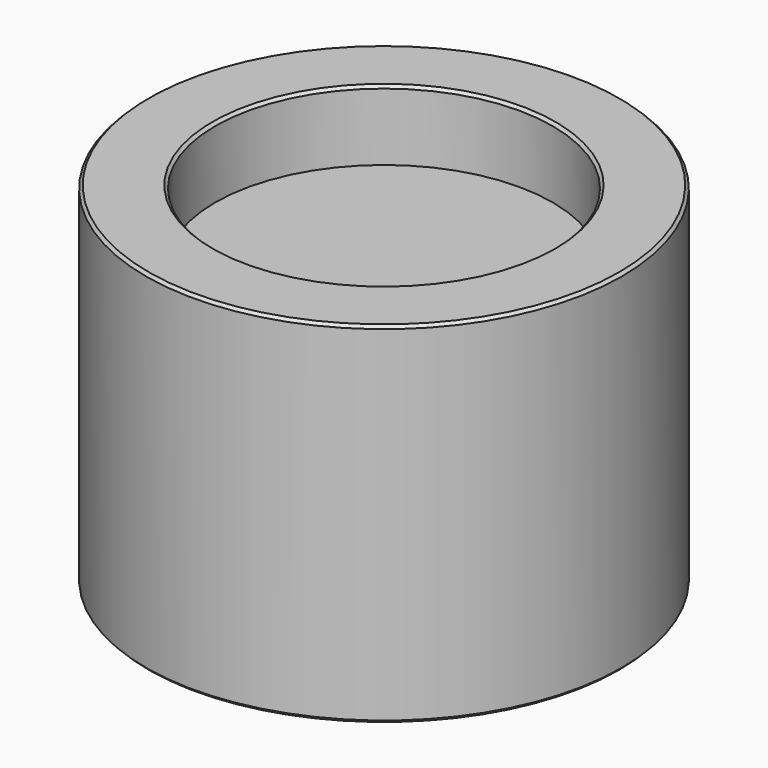
from build123d import *

# Parameters (mm, degrees)
F0_R     = 17
F1_DEPTH = 25
F3_D     = 9
F3_DEPTH = 17
F3_TIP   = 2.7038727856
F4_R     = 12.05
F5_DEPTH = 5
F6_SIZE  = 0.2


with BuildPart() as f1:
    # F0 (on Top) → F1 (new body)
    with BuildSketch(Plane.XY):
        Circle(F0_R)
    extrude(amount=F1_DEPTH)

    # F3
    with Locations(Plane(origin=(0, 0, 0), x_dir=(1, 0, 0), z_dir=(0, 0, -1))):
        with Locations((0, 0)):
            Hole(F3_D / 2, depth=F3_DEPTH)
            with Locations((0, 0, -(F3_DEPTH + F3_TIP / 2))):  # 118° drill point
                Cone(0, F3_D / 2, F3_TIP, mode=Mode.SUBTRACT)

    # F4 (on face) → F5 (cut)
    with BuildSketch(Plane.XY.offset(25)):
        Circle(F4_R)
    extrude(amount=-F5_DEPTH, mode=Mode.SUBTRACT)

    # F6
    f6_edges = [f1.edges().sort_by_distance(p)[0] for p in [
        (-17, 0, 25),
        (-12.05, 0, 25),
        (-17, 0, 0),
        (-4.5, 0, 0),
    ]]
    chamfer(f6_edges, length=F6_SIZE)


solid = f1.part
